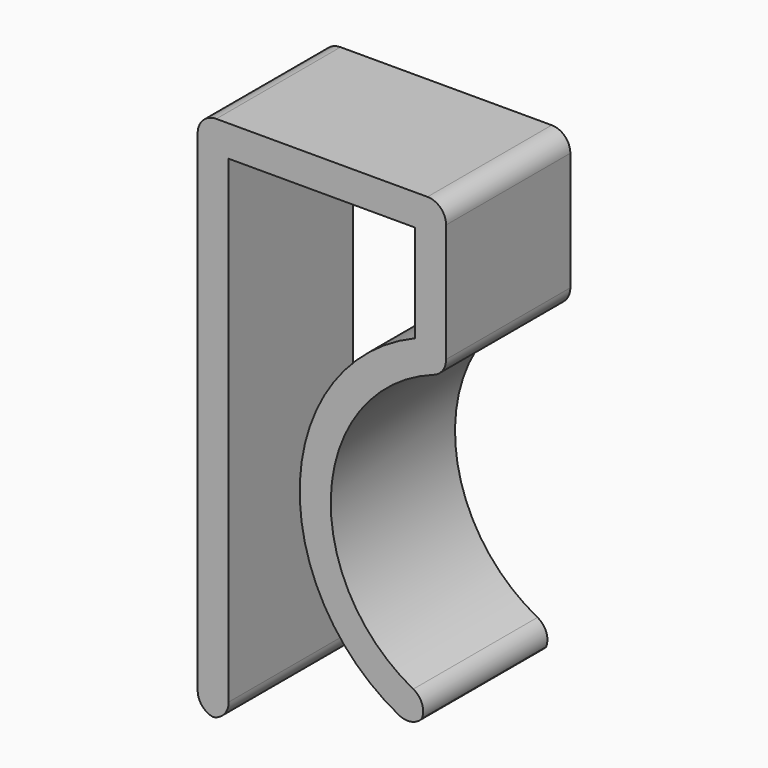
from build123d import *

# Parameters (mm, degrees)
F1_DEPTH    = 25
F2_T1_DEPTH = 40
F2_T3_DEPTH = 36.0263819839
F2_T5_DEPTH = 41.8333819759
F2_T7_DEPTH = 39.2479422715


# Not quite as in the source:
# - a fillet or chamfer that OpenCascade refuses, or shapes differently, is made with other operations: its cross-section is extruded or revolved along the edge and cut away or added


with BuildPart() as f1:
    # F0 (on Front) → F1 (new body)
    with BuildSketch(Plane.XZ):
        with BuildLine():
            Line((-5, -80), (0, -80))
            Line((0, -80), (0, 0))
            Line((0, 0), (30, 0))
            Line((30, 0), (30, -15.6914651025))
            ThreePointArc((30, -15.6914651025), (11.4304994047, -43.4285104275), (30, -71.1655557525))
            Line((30, -71.1655557525), (32.6106493124, -66.8210358224))
            ThreePointArc((32.6106493124, -66.8210358224), (16.4620002863, -42.1738982265), (35, -19.26968849))
            Line((35, -19.26968849), (35, 5))
            Line((35, 5), (-5, 5))
            Line((-5, 5), (-5, -80))
        make_face()
    extrude(amount=F1_DEPTH)

    # F2: fillet of radius 3 on 7 edges, made by hand

    # F2_s2 → F2_t1 (cut)
    with BuildSketch(Plane.XZ.offset(-7.5)):
        with BuildLine():
            ThreePointArc((35, 2), (34.1213203436, 4.1213203436), (32, 5))
            Line((32, 5), (35, 5))
            Line((35, 5), (35, 2))
        make_face()
        with BuildLine():
            ThreePointArc((-3, -80), (-0.8786796564, -79.1213203436), (0, -77))
            Line((0, -77), (0, -80))
            Line((0, -80), (-3, -80))
        make_face()
        with BuildLine():
            ThreePointArc((-2, -80), (-4.1213203436, -79.1213203436), (-5, -77))
            Line((-5, -77), (-5, -80))
            Line((-5, -80), (-2, -80))
        make_face()
        with BuildLine():
            ThreePointArc((-2, 5), (-4.1213203436, 4.1213203436), (-5, 2))
            Line((-5, 2), (-5, 5))
            Line((-5, 5), (-2, 5))
        make_face()
    extrude(amount=F2_T1_DEPTH, mode=Mode.SUBTRACT)

    # F2_s4 → F2_t3 (cut)
    with BuildSketch(Plane.XZ.offset(-5.513190992)):
        with BuildLine():
            ThreePointArc((33.0104106505, -19.8891369147), (34.4526752691, -18.7919490752), (35, -17.0644120932))
            Line((35, -17.0644120932), (35, -19.26968849))
            ThreePointArc((35, -19.26968849), (33.9987485172, -19.5586742582), (33.0104106505, -19.8891369147))
        make_face()
    extrude(amount=F2_T3_DEPTH, mode=Mode.SUBTRACT)

    # F2_s6 → F2_t5 (cut)
    with BuildSketch(Plane.XZ.offset(-8.416690988)):
        with BuildLine():
            ThreePointArc((30.8765859694, -69.7067825667), (31.1957188728, -67.3587557485), (29.7114248515, -65.5116101106))
            ThreePointArc((29.7114248515, -65.5116101106), (31.1401881693, -66.212484942), (32.6106493124, -66.8210358224))
            Line((32.6106493124, -66.8210358224), (30.8765859694, -69.7067825667))
        make_face()
    extrude(amount=F2_T5_DEPTH, mode=Mode.SUBTRACT)

    # F2_s8 → F2_t7 (cut)
    with BuildSketch(Plane.XZ.offset(-7.1239711357)):
        with BuildLine():
            ThreePointArc((27.4198994503, -69.9559130315), (29.6266357528, -70.1929626749), (31.39240951, -68.8483732652))
            Line((31.39240951, -68.8483732652), (30, -71.1655557525))
            ThreePointArc((30, -71.1655557525), (28.695579184, -70.5913859559), (27.4198994503, -69.9559130315))
        make_face()
    extrude(amount=F2_T7_DEPTH, mode=Mode.SUBTRACT)


solid = f1.part
